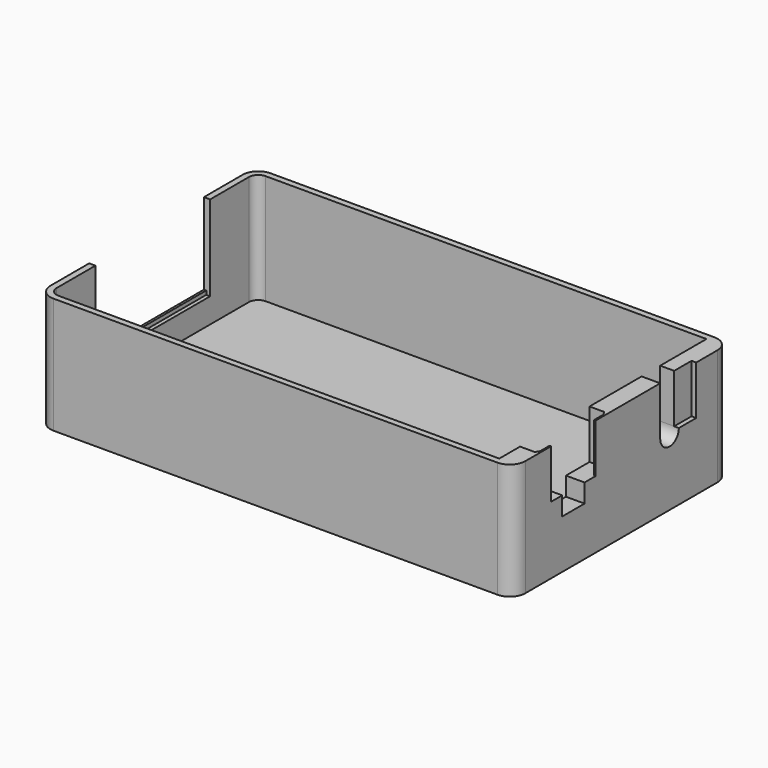
from build123d import *

# Parameters (mm, degrees)
F1_W      = 155.575
F1_H      = 88.9
F2_DEPTH  = 38.1
F3_R      = 5.08
F4_T      = -2.032
F5_W      = 46.99
F5_H      = 26.67
F6_DEPTH  = 2.032
F7_W      = 1.27
F7_H      = 46.99
F8_DEPTH  = 1.27
F11_DEPTH = 36.068
F12_DEPTH = 6.096
F13_W     = 1.524
F13_H     = 7.112
F14_DEPTH = 16.002
F16_DEPTH = 16.002


# Not quite as in the source:
# - a variable given as a bare number and used for a length is read in inches; the dataset says mm whatever the document's units were


with BuildPart() as f2:
    # F1 (on Top) → F2 (new body)
    with BuildSketch(Plane.XY):
        Rectangle(F1_W, F1_H)
    extrude(amount=F2_DEPTH)

    # F3
    f3_edges = [f2.edges().sort_by_distance(p)[0] for p in [
        (77.7875, -44.45, 19.05),
        (-77.7875, -44.45, 19.05),
        (77.7875, 44.45, 19.05),
        (-77.7875, 44.45, 19.05),
    ]]
    fillet(f3_edges, radius=F3_R)

    # F4
    f4_openings = [f2.faces().sort_by_distance(p)[0] for p in [
        (0, 0, 38.1),
    ]]
    offset(amount=F4_T, openings=f4_openings)

    # F5 (on face) → F6 (cut, through all)
    with BuildSketch(Plane(origin=(-77.7875, 0, 0), x_dir=(0, -1, 0), z_dir=(-1, 0, 0))):
        with Locations((0, 24.765)):
            Rectangle(F5_W, F5_H)
    extrude(amount=-F6_DEPTH, mode=Mode.SUBTRACT)

    # F7 (on face) → F8 (cut)
    with BuildSketch(Plane.XY.offset(11.43)):
        with Locations((-76.3905, 0)):
            Rectangle(F7_W, F7_H)
    extrude(amount=-F8_DEPTH, mode=Mode.SUBTRACT)

    # F10 (on face) → F11 (join, through all)
    with BuildSketch(Plane.XY.offset(2.032)):
        with BuildLine():
            ThreePointArc((72.7075, -42.418), (74.8627614691, -41.5252614691), (75.7555, -39.37))
            Line((75.7555, -39.37), (75.7555, 39.37))
            ThreePointArc((75.7555, 39.37), (74.8627614691, 41.5252614691), (72.7075, 42.418))
            Line((72.7075, 42.418), (71.6915, 42.418))
            Line((71.6915, 42.418), (71.6915, -42.418))
            Line((71.6915, -42.418), (72.7075, -42.418))
        make_face()
    extrude(amount=F11_DEPTH)

    # F9 (on face) → F12 (cut, through all)
    with BuildSketch(Plane.YZ.offset(77.7875)):
        Polygon((-10.541, 38.1), (-28.829, 38.1), (-28.829, 22.098), (-24.257, 22.098), (-24.257, 16.002), (-15.113, 16.002), (-15.113, 22.098), (-10.541, 22.098), align=None)
        with BuildLine():
            Line((23.495, 38.1), (15.875, 38.1))
            Line((15.875, 38.1), (15.875, 22.098))
            ThreePointArc((15.875, 22.098), (19.685, 18.288), (23.495, 22.098))
            Line((23.495, 22.098), (23.495, 38.1))
        make_face()
    extrude(amount=-F12_DEPTH, mode=Mode.SUBTRACT)

    # F13 (on face) → F14 (cut)
    with BuildSketch(Plane.XY.offset(38.1)):
        with Locations((77.0255, 27.051)):
            Rectangle(F13_W, F13_H)
    extrude(amount=-F14_DEPTH, mode=Mode.SUBTRACT)

    # F15 (on face) → F16 (cut, through all)
    with BuildSketch(Plane.XY.offset(38.1)):
        Polygon((77.2795, -32.639), (77.2795, -28.829), (71.6915, -28.829), (71.6915, -33.909), (76.5175, -33.909), align=None)
        Polygon((71.6915, -10.541), (77.2795, -10.541), (77.2795, -6.731), (76.5175, -5.461), (71.6915, -5.461), align=None)
    extrude(amount=-F16_DEPTH, mode=Mode.SUBTRACT)


solid = f2.part
